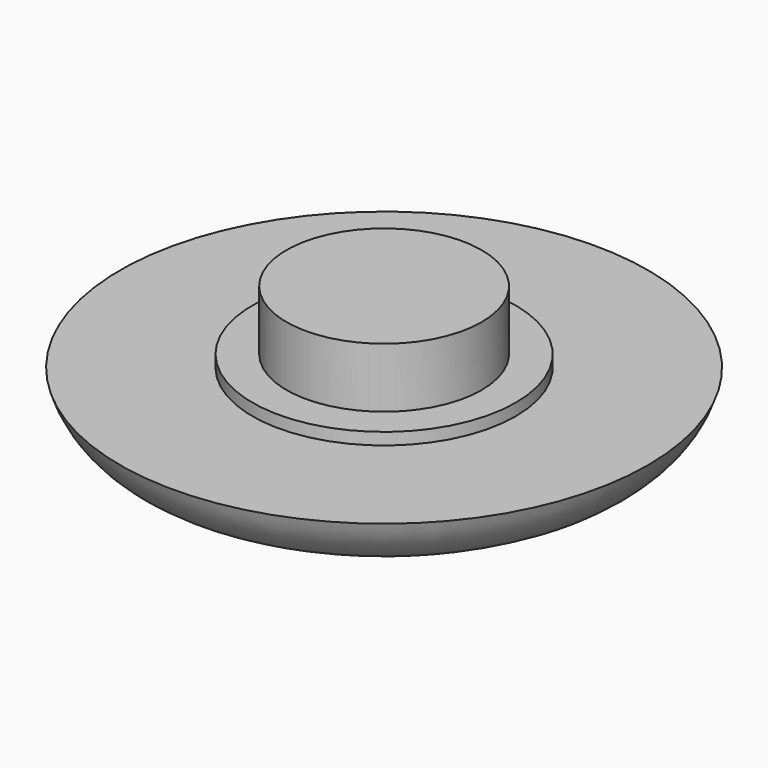
from build123d import *

# Parameters (mm, degrees)
F0_R     = 11.025
F0_R_2   = 5.5
F1_DEPTH = 2.5
F0_R_3   = 4.075
F2_DEPTH = 3
F3_DEPTH = 5.5


# Not quite as in the source:
# - a fillet or chamfer that OpenCascade refuses, or shapes differently, is made with other operations: its cross-section is extruded or revolved along the edge and cut away or added


with BuildPart() as f1:
    # F0 (on Top) → F1 (new body)
    with BuildSketch(Plane.XY):
        Circle(F0_R)
        Circle(F0_R_2, mode=Mode.SUBTRACT)
    extrude(amount=F1_DEPTH)

    # F0 (on Top) → F2 (join)
    with BuildSketch(Plane.XY):
        Circle(F0_R_2)
        Circle(F0_R_3, mode=Mode.SUBTRACT)
    extrude(amount=F2_DEPTH)

    # F0 (on Top) → F3 (join)
    with BuildSketch(Plane.XY):
        Circle(F0_R_3)
    extrude(amount=F3_DEPTH)

    # F4: fillet of radius 3.5 on 1 edges, made by hand

    # F4_s1 → F4_t2 (revolve, cut)
    with BuildSketch(Plane.XZ):
        with BuildLine():
            ThreePointArc((11.025, 2.5), (9.7625481001, 0.6937569599), (7.6708980338, 0))
            Line((7.6708980338, 0), (11.025, 0))
            Line((11.025, 0), (11.025, 2.5))
        make_face()
    revolve(axis=Axis((0, 0, 0), (0, 0, 1)), mode=Mode.SUBTRACT)


solid = f1.part
